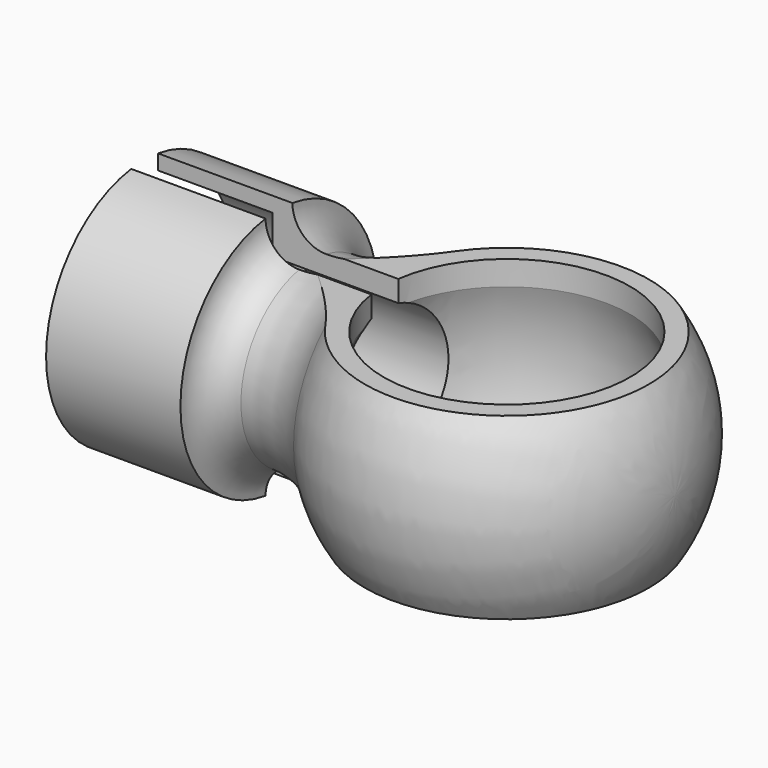
from build123d import *

# Parameters (mm, degrees)
F3_DEPTH = 35.350352
F5_DEPTH = 20
F8_R     = 2.99999


# Not quite as in the source:
# - a fillet or chamfer is up to 0.001 mm smaller than in the source, because OpenCascade refuses the exact size
# - ends of sketch curves that miss each other by under 0.0002 mm in the source are joined


with BuildPart() as f1:
    # F0 (on Front) → F1 (revolve)
    with BuildSketch(Plane.XZ):
        with BuildLine():
            Line((4.524581, 0.442101), (26.091657, 0.442101))
            ThreePointArc((26.091657, 0.442101), (16.959188, 14.246886), (0.682046, 11.242101))
            ThreePointArc((0.682046, 11.242101), (-2.516037, 9.168482), (-6.257695, 8.442101))
            Line((-6.257695, 8.442101), (-9.257695, 8.442101))
            Line((-9.257695, 8.442101), (-9.257695, 11.442101))
            Line((-9.257695, 11.442101), (-21.257695, 11.442101))
            Line((-21.257695, 11.442101), (-21.257695, 10.113103))
            Line((-21.257695, 10.113103), (-11.030108, 10.113103))
            Line((-11.030108, 10.113103), (-11.030108, 6.723208))
            Line((-11.030108, 6.723208), (4.524581, 6.723208))
            Line((4.524581, 6.723208), (4.524581, 0.442101))
        make_face()
    revolve(axis=Axis((2.416981, 0, 0.442101), (-1, 0, 0)))

    # F2 (on face) → F3 (cut, through all)
    with BuildSketch(Plane.YZ.offset(-9.257695)):
        with BuildLine():
            Line((33.242781, -24.965025), (33.242781, -7.557899))
            Line((33.242781, -7.557899), (7.549834, -7.557899))
            ThreePointArc((7.549834, -7.557899), (0, -10.557899), (-7.549834, -7.557899))
            Line((-7.549834, -7.557899), (-33.242781, -7.557899))
            Line((-33.242781, -7.557899), (-36.838822, -7.557899))
            Line((-36.838822, -7.557899), (-36.838822, -24.965025))
            Line((-36.838822, -24.965025), (33.242781, -24.965025))
        make_face()
        with BuildLine():
            Line((7.549834, 8.442101), (33.242781, 8.442101))
            Line((33.242781, 8.442101), (33.242781, 29.21157))
            Line((33.242781, 29.21157), (-51.441289, 29.21157))
            Line((-51.441289, 29.21157), (-51.441289, 8.442101))
            Line((-51.441289, 8.442101), (-33.242781, 8.442101))
            Line((-33.242781, 8.442101), (-7.549834, 8.442101))
            ThreePointArc((-7.549834, 8.442101), (0, 11.442101), (7.549834, 8.442101))
        make_face()
        with BuildLine():
            ThreePointArc((-7.549834, -7.557899), (0, -10.557899), (7.549834, -7.557899))
            Line((7.549834, -7.557899), (0, -7.557899))
            Line((0, -7.557899), (-7.549834, -7.557899))
        make_face()
        with BuildLine():
            Line((0, 8.442101), (7.549834, 8.442101))
            ThreePointArc((7.549834, 8.442101), (0, 11.442101), (-7.549834, 8.442101))
            Line((-7.549834, 8.442101), (0, 8.442101))
        make_face()
    extrude(amount=F3_DEPTH, mode=Mode.SUBTRACT)

    # F4 (on face) → F5 (cut, symmetric)
    with BuildSketch(Plane(origin=(0, 0, -7.557899), x_dir=(1, 0, 0), z_dir=(0, 0, -1))):
        with BuildLine():
            Line((-4.593732, -1.5), (0.19441, -1.5))
            ThreePointArc((0.19441, -1.5), (22.091657, 0), (0.19441, 1.5))
            Line((0.19441, 1.5), (-4.593732, 1.5))
            add(Edge.make_bspline(
                [(-4.593732, 1.5), (-4.766224, 1.342053), (-4.939191, 1.184637), (-5.112549, 1.027662), (-5.286215, 0.871035), (-5.522815, 0.658273), (-5.585554, 0.601915), (-5.648318, 0.545587), (-5.711103, 0.489282), (-5.813747, 0.397293), (-5.853595, 0.361596), (-5.893449, 0.325906), (-5.933308, 0.290222), (-5.994638, 0.235329), (-6.016107, 0.216117), (-6.037577, 0.196905), (-6.059048, 0.177694), (-6.115953, 0.126783), (-6.151387, 0.095086), (-6.186822, 0.06339), (-6.222258, 0.031695), (-6.257694, 0)],
                knots=[0.777274, 0.777274, 0.777274, 0.777274, 0.777274, 0.777274, 0.893527, 0.893527, 0.893527, 0.893527, 0.93545, 0.93545, 0.93545, 0.93545, 0.962045, 0.962045, 0.962045, 0.962045, 0.976367, 0.976367, 0.976367, 0.976367, 1, 1, 1, 1, 1, 1], degree=5))
            add(Edge.make_bspline(
                [(-4.593732, -1.5), (-4.766224, -1.342053), (-4.939191, -1.184637), (-5.112549, -1.027662), (-5.286215, -0.871035), (-5.522815, -0.658273), (-5.585554, -0.601915), (-5.648318, -0.545587), (-5.711103, -0.489282), (-5.813747, -0.397293), (-5.853595, -0.361596), (-5.893449, -0.325906), (-5.933308, -0.290222), (-5.994638, -0.235329), (-6.016107, -0.216117), (-6.037577, -0.196905), (-6.059048, -0.177694), (-6.115953, -0.126783), (-6.151387, -0.095086), (-6.186822, -0.06339), (-6.222258, -0.031695), (-6.257694, 0)],
                knots=[0.777274, 0.777274, 0.777274, 0.777274, 0.777274, 0.777274, 0.893527, 0.893527, 0.893527, 0.893527, 0.93545, 0.93545, 0.93545, 0.93545, 0.962045, 0.962045, 0.962045, 0.962045, 0.976367, 0.976367, 0.976367, 0.976367, 1, 1, 1, 1, 1, 1], degree=5))
        make_face()
        with BuildLine():
            Line((-31.996746, -1.5), (-4.593732, -1.5))
            add(Edge.make_bspline(
                [(-4.593732, -1.5), (-4.766224, -1.342053), (-4.939191, -1.184637), (-5.112549, -1.027662), (-5.286215, -0.871035), (-5.522815, -0.658273), (-5.585554, -0.601915), (-5.648318, -0.545587), (-5.711103, -0.489282), (-5.813747, -0.397293), (-5.853595, -0.361596), (-5.893449, -0.325906), (-5.933308, -0.290222), (-5.994638, -0.235329), (-6.016107, -0.216117), (-6.037577, -0.196905), (-6.059048, -0.177694), (-6.115953, -0.126783), (-6.151387, -0.095086), (-6.186822, -0.06339), (-6.222258, -0.031695), (-6.257694, 0)],
                knots=[0.777274, 0.777274, 0.777274, 0.777274, 0.777274, 0.777274, 0.893527, 0.893527, 0.893527, 0.893527, 0.93545, 0.93545, 0.93545, 0.93545, 0.962045, 0.962045, 0.962045, 0.962045, 0.976367, 0.976367, 0.976367, 0.976367, 1, 1, 1, 1, 1, 1], degree=5))
            add(Edge.make_bspline(
                [(-4.593732, 1.5), (-4.766224, 1.342053), (-4.939191, 1.184637), (-5.112549, 1.027662), (-5.286215, 0.871035), (-5.522815, 0.658273), (-5.585554, 0.601915), (-5.648318, 0.545587), (-5.711103, 0.489282), (-5.813747, 0.397293), (-5.853595, 0.361596), (-5.893449, 0.325906), (-5.933308, 0.290222), (-5.994638, 0.235329), (-6.016107, 0.216117), (-6.037577, 0.196905), (-6.059048, 0.177694), (-6.115953, 0.126783), (-6.151387, 0.095086), (-6.186822, 0.06339), (-6.222258, 0.031695), (-6.257694, 0)],
                knots=[0.777274, 0.777274, 0.777274, 0.777274, 0.777274, 0.777274, 0.893527, 0.893527, 0.893527, 0.893527, 0.93545, 0.93545, 0.93545, 0.93545, 0.962045, 0.962045, 0.962045, 0.962045, 0.976367, 0.976367, 0.976367, 0.976367, 1, 1, 1, 1, 1, 1], degree=5))
            Line((-4.593732, 1.5), (-31.996746, 1.5))
            Line((-31.996746, 1.5), (-31.996746, -1.5))
        make_face()
    extrude(amount=F5_DEPTH, both=True, mode=Mode.SUBTRACT)

    # F6 (on Front) → F7 (revolve, cut)
    with BuildSketch(Plane.XZ):
        with BuildLine():
            Line((0.19441, -5.657269), (0.19441, 6.541471))
            ThreePointArc((0.19441, 6.541471), (-0.919143, 0.442101), (0.19441, -5.657269))
        make_face()
    revolve(axis=Axis((11.091657, 0, 0.442101), (0, 0, 1)), mode=Mode.SUBTRACT)

    # F8 (radius 3 in the source; OpenCascade refuses exactly that, so slightly less here)
    f8_edges = [f1.edges().sort_by_distance(p)[0] for p in [
        (-9.257695, -8, 0.442101),
        (-9.257695, 8, 0.442101),
    ]]
    fillet(f8_edges, radius=F8_R)


solid = f1.part
